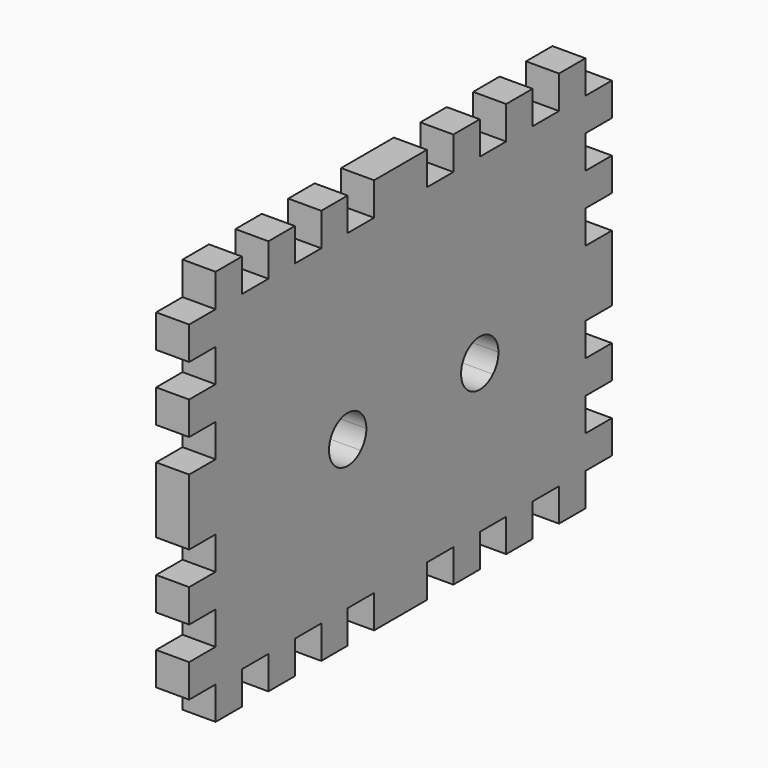
from build123d import *

# Parameters (mm, degrees)
F1_DEPTH = 6.35
F2_W     = 6.35
F2_H     = 6.35
F3_DEPTH = 6.351


with BuildPart() as f1:
    # F0 (on Right) → F1 (new body)
    with BuildSketch(Plane.YZ):
        Polygon((-38.1, 38.1), (-44.45, 38.1), (-44.45, 31.75), (-50.8, 31.75), (-50.8, 25.4), (-44.45, 25.4), (-44.45, 19.05), (-50.8, 19.05), (-50.8, 12.7), (-44.45, 12.7), (-44.45, 6.35), (-50.8, 6.35), (-50.8, 0), (-50.8, -6.35), (-44.45, -6.35), (-44.45, -12.7), (-50.8, -12.7), (-50.8, -19.05), (-44.45, -19.05), (-44.45, -25.4), (-50.8, -25.4), (-50.8, -31.75), (-44.45, -31.75), (-44.45, -38.1), (-38.1, -38.1), (-38.1, -31.75), (-31.75, -31.75), (-31.75, -38.1), (-25.4, -38.1), (-25.4, -31.75), (-19.05, -31.75), (-19.05, -38.1), (-12.7, -38.1), (-12.7, -31.75), (-6.35, -31.75), (-6.35, -38.1), (0, -38.1), (6.35, -38.1), (6.35, -31.75), (12.7, -31.75), (12.7, -38.1), (19.05, -38.1), (19.05, -31.75), (25.4, -31.75), (25.4, -38.1), (31.75, -38.1), (31.75, -31.75), (38.1, -31.75), (38.1, -38.1), (44.45, -38.1), (44.45, -31.75), (50.8, -31.75), (50.8, -25.4), (44.45, -25.4), (44.45, -19.05), (50.8, -19.05), (50.8, -12.7), (44.45, -12.7), (44.45, -6.35), (50.8, -6.35), (50.8, 0), (50.8, 6.35), (44.45, 6.35), (44.45, 12.7), (50.8, 12.7), (50.8, 19.05), (44.45, 19.05), (44.45, 25.4), (50.8, 25.4), (50.8, 31.75), (44.45, 31.75), (44.45, 38.1), (38.1, 38.1), (38.1, 31.75), (31.75, 31.75), (31.75, 38.1), (25.4, 38.1), (25.4, 31.75), (19.05, 31.75), (19.05, 38.1), (12.7, 38.1), (12.7, 31.75), (6.35, 31.75), (6.35, 38.1), (0, 38.1), (-6.35, 38.1), (-6.35, 31.75), (-12.7, 31.75), (-12.7, 38.1), (-19.05, 38.1), (-19.05, 31.75), (-25.4, 31.75), (-25.4, 38.1), (-31.75, 38.1), (-31.75, 31.75), (-38.1, 31.75), align=None)
    extrude(amount=F1_DEPTH)

    # F2 (on face) → F3 (cut, through all)
    with BuildSketch(Plane.YZ.offset(6.35)):
        with BuildLine():
            ThreePointArc((-15.875, -6.35), (-12.7, -7.6651280605), (-9.525, -6.35))
            Line((-9.525, -6.35), (-15.875, -6.35))
        make_face()
        Polygon((-15.875, -6.35), (-9.525, -6.35), (-9.525, -3.175), (-9.525, 0), (-15.875, 0), align=None)
        with BuildLine():
            Line((-9.525, -3.175), (-9.525, -6.35))
            ThreePointArc((-9.525, -6.35), (-8.5516625865, -4.893297618), (-8.2098719395, -3.175))
            ThreePointArc((-8.2098719395, -3.175), (-8.5516625865, -1.456702382), (-9.525, 0))
            Line((-9.525, 0), (-9.525, -3.175))
        make_face()
        with BuildLine():
            ThreePointArc((-15.875, 0), (-17.1901280605, -3.175), (-15.875, -6.35))
            Line((-15.875, -6.35), (-15.875, 0))
        make_face()
        with BuildLine():
            Line((-15.875, 0), (-9.525, 0))
            ThreePointArc((-9.525, 0), (-12.7, 1.3151280605), (-15.875, 0))
        make_face()
        with BuildLine():
            ThreePointArc((22.225, 0), (19.05, 1.3151280605), (15.875, 0))
            Line((15.875, 0), (22.225, 0))
        make_face()
        with Locations((19.05, -3.175)):
            Rectangle(F2_W, F2_H)
        with BuildLine():
            Line((15.875, -6.35), (15.875, 0))
            ThreePointArc((15.875, 0), (14.5598719395, -3.175), (15.875, -6.35))
        make_face()
        with BuildLine():
            ThreePointArc((23.5401280605, -3.175), (23.1983374135, -1.456702382), (22.225, 0))
            Line((22.225, 0), (22.225, -6.35))
            ThreePointArc((22.225, -6.35), (23.1983374135, -4.893297618), (23.5401280605, -3.175))
        make_face()
        with BuildLine():
            Line((22.225, -6.35), (15.875, -6.35))
            ThreePointArc((15.875, -6.35), (19.05, -7.6651280605), (22.225, -6.35))
        make_face()
    extrude(amount=-F3_DEPTH, mode=Mode.SUBTRACT)


solid = f1.part
